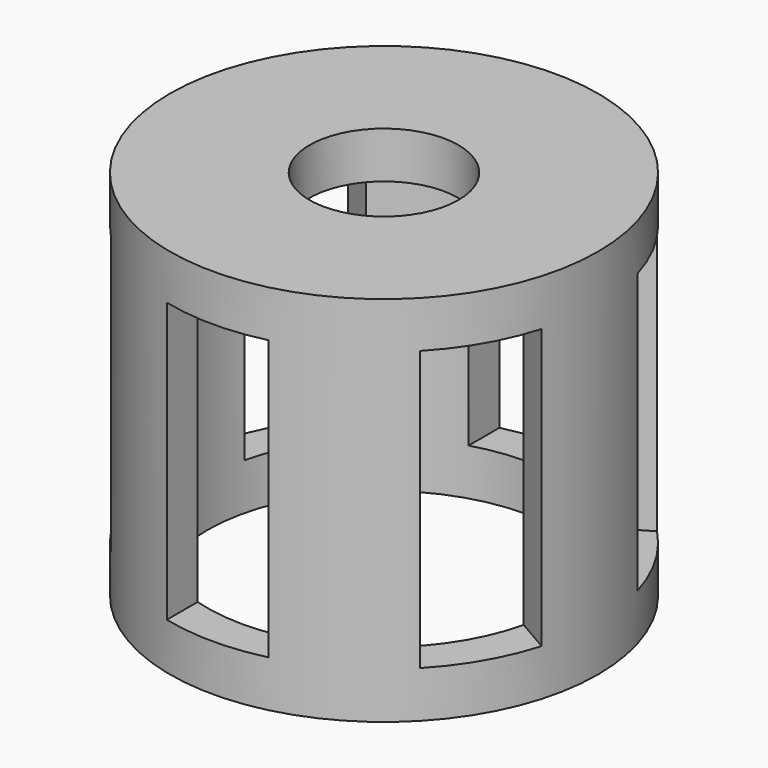
from build123d import *

# Parameters (mm, degrees)
F0_R     = 11.5
F0_R_2   = 9.5
F1_DEPTH = 10
F2_W     = 5.4703750648
F2_H     = 6.3438538521
F3_DEPTH = 7.5
F4_R     = 4
F5_DEPTH = 2.5


with BuildPart() as f1:
    # F0 (on Top) → F1 (new body, symmetric)
    with BuildSketch(Plane.XY):
        Circle(F0_R)
        Circle(F0_R_2, mode=Mode.SUBTRACT)
    extrude(amount=F1_DEPTH, both=True)

    # F2 (on Top) → F3 (cut, symmetric)
    with BuildSketch(Plane.XY):
        with Locations((0, 9.139645283)):
            Rectangle(F2_W, F2_H)
        Polygon((-3.8006019335, 5.3526010656), (-9.2945405273, 8.5245279917), (-12.0297280597, 3.7870442173), (-6.5357894659, 0.6151172913), align=None)
        Polygon((-6.5357894659, -0.6151172913), (-12.0297280597, -3.7870442173), (-9.2945405273, -8.5245279917), (-3.8006019335, -5.3526010656), align=None)
        with Locations((0, -9.139645283)):
            Rectangle(F2_W, F2_H)
        Polygon((3.8006019335, -5.3526010656), (9.2945405273, -8.5245279917), (12.0297280597, -3.7870442173), (6.5357894659, -0.6151172913), align=None)
        Polygon((6.5357894659, 0.6151172913), (12.0297280597, 3.7870442173), (9.2945405273, 8.5245279917), (3.8006019335, 5.3526010656), align=None)
    extrude(amount=F3_DEPTH, both=True, mode=Mode.SUBTRACT)

    # F4 (on face) → F5 (join, through all)
    with BuildSketch(Plane(origin=(0, 0, 7.5), x_dir=(1, 0, 0), z_dir=(0, 0, -1))):
        with BuildLine():
            ThreePointArc((-2.7351875324, 9.0977331881), (-5.6685852928, -7.6234598955), (9.5, 0))
            ThreePointArc((9.5, 0), (7.6234598955, 5.6685852928), (2.7351875324, 9.0977331881))
            ThreePointArc((2.7351875324, 9.0977331881), (0, 9.5), (-2.7351875324, 9.0977331881))
        make_face()
        Circle(F4_R, mode=Mode.SUBTRACT)
    extrude(amount=-F5_DEPTH)


solid = f1.part
